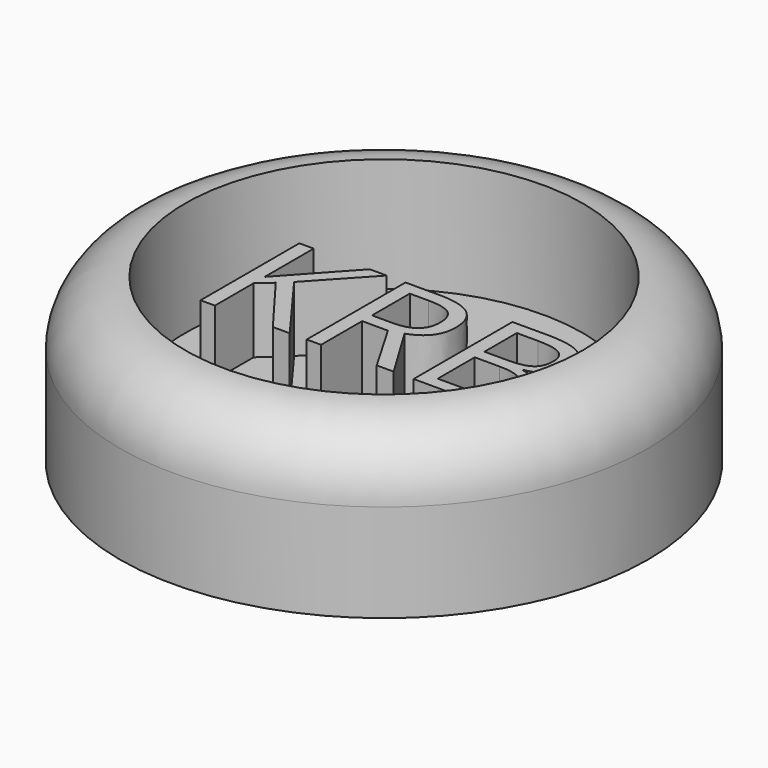
from build123d import *

# Parameters (mm, degrees)
F0_R         = 20.5777343559
F1_DEPTH     = 12.7
F5_R         = 5.08
F6_DEPTH     = 8.89
F7_TEXT_SIZE = 13.4757057013
F8_DEPTH     = 5.08


# Not quite as in the source:
# - the program builds the solid bodies; features that only make, move or delete a surface that nothing else refers to are left out
# - Text() gives the source's letters only with a copy of the font that has no kerning and outlines rounded to 1/6400 em; it was checked with that copy


with BuildPart() as f1:
    # F0 (on Top) → F1 (new body)
    with BuildSketch(Plane.XY):
        Circle(F0_R)
    extrude(amount=F1_DEPTH)

    # F5
    f5_edges = [f1.edges().sort_by_distance(p)[0] for p in [
        (-20.577734, 0, 12.7),
    ]]
    fillet(f5_edges, radius=F5_R)

    # F6 (cut): a face of the model
    f6_faces = [f1.faces().sort_by_distance(p)[0] for p in [
        (0, 0, 12.7),
    ]]
    extrude(f6_faces, amount=-F6_DEPTH, mode=Mode.SUBTRACT)

    # F7 (on face) → F8 (join)
    with BuildSketch(Plane.XY.offset(3.81)):
        with Locations((-12.6806749031, -3.6679909099)):
            Text('KRB', F7_TEXT_SIZE, font='Open Sans', text_align=(TextAlign.LEFT, TextAlign.BOTTOM))
    extrude(amount=F8_DEPTH)


solid = f1.part
